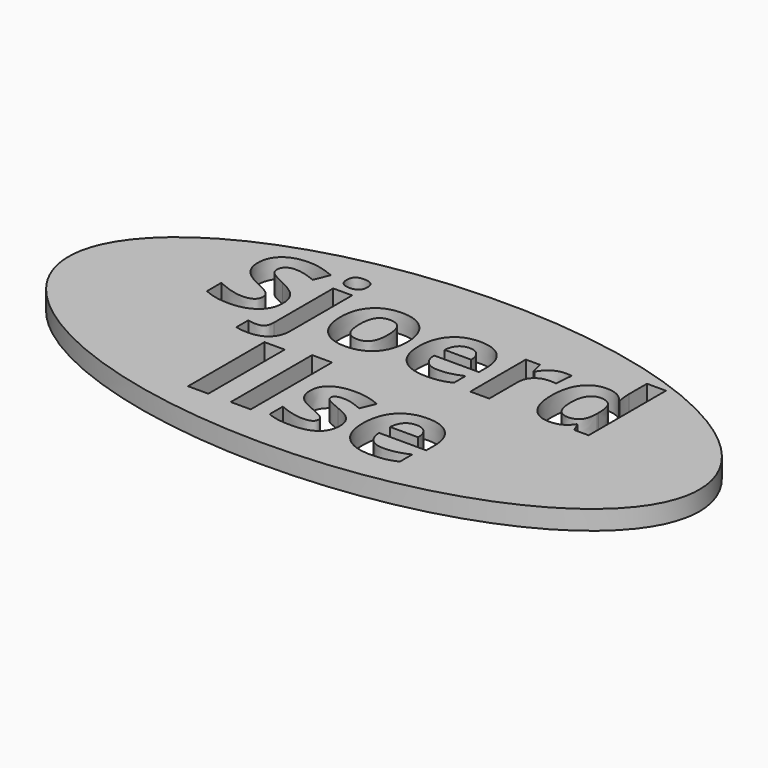
from build123d import *

# Parameters (mm, degrees)
F2_DEPTH       = 8
F0_TEXT_SIZE   = 52.7777777778
F0_TEXT_SIZE_2 = 55.5555555556
F3_DEPTH       = 25


# Not quite as in the source:
# - Text() gives the source's letters only with a copy of the font that has no kerning and outlines rounded to 1/6400 em; it was checked with that copy


with BuildPart() as f2:
    # F1 (on Top) → F2 (new body)
    with BuildSketch(Plane.XY):
        with BuildLine():
            add(Edge.make_bspline(
                [(132.7215698144, 20.5380003899), (132.7215698144, 129.5331309021), (-63.7147827454, 75.035565646), (-260.1511353052, 20.5380003899), (-63.7147827454, -33.9595648661), (132.7215698144, -88.4571301222), (132.7215698144, 20.5380003899)],
                knots=[0, 0, 0, 2.0943951024, 2.0943951024, 4.1887902048, 4.1887902048, 6.2831853072, 6.2831853072, 6.2831853072], degree=2, weights=[1, 0.5, 1, 0.5, 1, 0.5, 1]))
        make_face()
    extrude(amount=F2_DEPTH)

    # F0 (on Top) → F3 (cut)
    with BuildSketch(Plane.XY):
        with Locations((-81.4194516095, 27.8495201462)):
            Text('Sjoerd', F0_TEXT_SIZE, font='Open Sans', font_style=FontStyle.BOLD, text_align=(TextAlign.LEFT, TextAlign.BOTTOM))
        with Locations((-47.0566043873, -26.379172298)):
            Text('Ilse', F0_TEXT_SIZE_2, font='Open Sans', font_style=FontStyle.BOLD, text_align=(TextAlign.LEFT, TextAlign.BOTTOM))
    extrude(amount=F3_DEPTH, mode=Mode.SUBTRACT)


solid = f2.part
